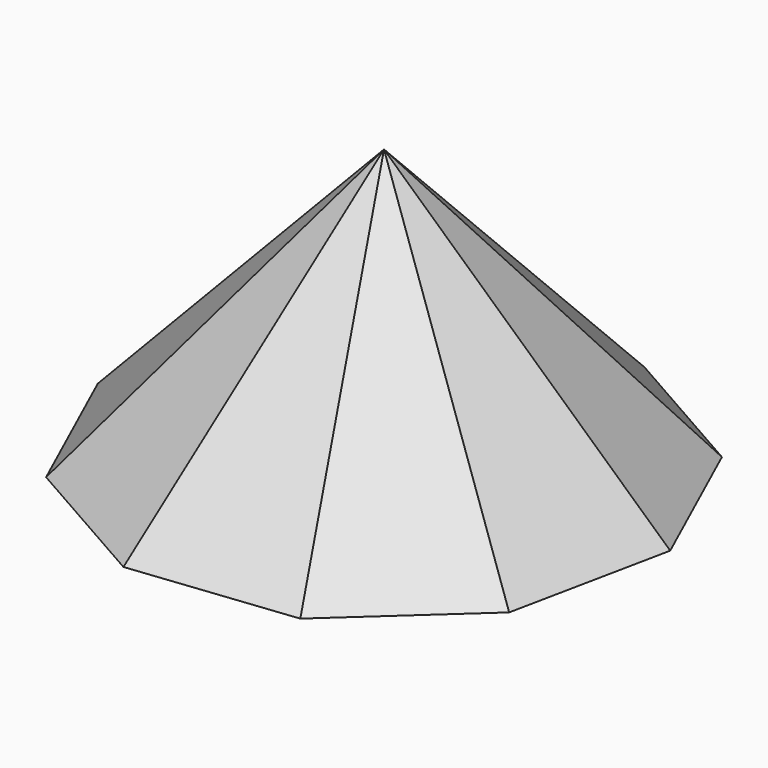
from build123d import *


# Not quite as in the source:
# - the program builds the solid bodies; features that only make, move or delete a surface that nothing else refers to are left out


with BuildPart() as f3:
    # F1 (on Top) → F3 section 0
    with BuildSketch(Plane.XY, mode=Mode.PRIVATE) as f3_s0:
        Polygon((-2039.0098238841, 1160.5409943), (-2331.7424803501, -259.6025167011), (-1733.8287623343, -1580.5866898873), (-473.651387779, -2297.8404697023), (967.4447180893, -2137.397290816), (2039.0098238841, -1160.5409943), (2331.7424803501, 259.6025167011), (1733.8287623343, 1580.5866898873), (473.651387779, 2297.8404697023), (-967.4447180893, 2137.397290816), align=None)
    loft([f3_s0.sketch, Vertex(0, 0, 2482)])


solid = f3.part
